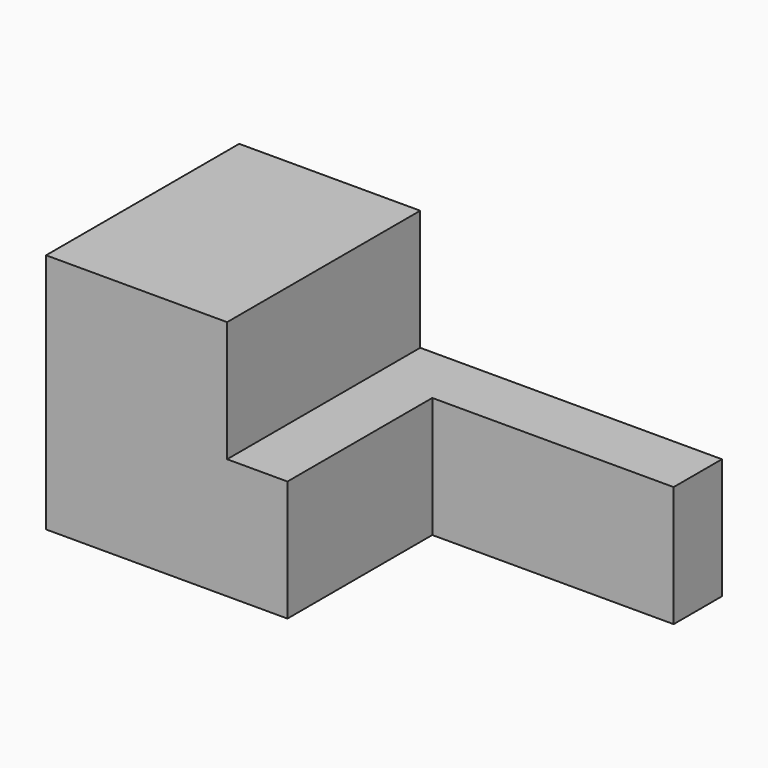
from build123d import *

# Parameters (mm, degrees)
F0_W     = 101.6
F0_H     = 76.2000028044
F1_DEPTH = 101.6
F2_W     = 50.8
F2_H     = 25.4
F3_DEPTH = 101.6
F4_W     = 50.8
F4_H     = 101.6
F5_DEPTH = 25.4
F6_ANGLE = 90
F7_ANGLE = -90


# Not quite as in the source:
# - a feature names something its author has since deleted; it is built from what else it names


with BuildPart() as f1:
    # F0 (on Top) → F1 (new body)
    with BuildSketch(Plane.XY):
        with Locations((-7.9828569114, 8.4364293143)):
            Rectangle(F0_W, F0_H)
    extrude(amount=F1_DEPTH)

    # F2 (on Top) → F3 (join)
    with BuildSketch(Plane.XY):
        with Locations((-33.3828569114, -42.3635720879)):
            Rectangle(F2_W, F2_H)
    extrude(amount=F3_DEPTH)

    # F4 (on Top) → F5 (join)
    with BuildSketch(Plane.XY):
        with Locations((-33.3828569114, -105.8635720879)):
            Rectangle(F4_W, F4_H)
    extrude(amount=F5_DEPTH)


with BuildPart() as f1_1:
    # F6: moved
    add(f1.part.rotate(Axis((-58.7828569114, -4.2635706857, 101.6), (0, -1, 0)), F6_ANGLE))


with BuildPart() as f1_2:
    # F7: moved
    add(f1_1.part.rotate(Axis((42.8171430886, -156.6635720879, 127), (0, 0, -1)), F7_ANGLE))


solid = f1_2.part
